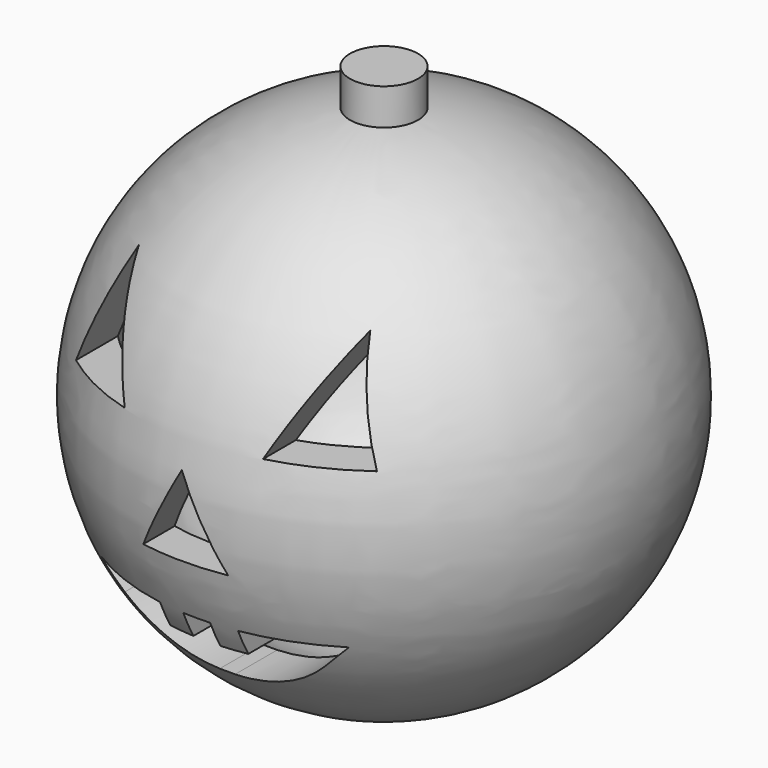
from build123d import *

# Parameters (mm, degrees)
F3_DEPTH = 50.8


# Not quite as in the source:
# - ends of sketch curves that miss each other by under 0.0002 mm in the source are joined


with BuildPart() as f1:
    # F0 (on Front) → F1 (revolve)
    with BuildSketch(Plane.XZ):
        with BuildLine():
            Line((-0.0036151696, -32.4747725203), (-0.0038838866, -38.0999998022))
            ThreePointArc((-0.0038838866, -38.0999998022), (38.0147276158, -2.5476258416), (5.0799988574, 37.7598146182))
            Line((5.0799988574, 37.7598146182), (5.0799988574, 43.18))
            Line((5.0799988574, 43.18), (-1.1426e-06, 43.18))
            Line((-1.1426e-06, 43.18), (-0.0005125311, 32.4747727174))
            ThreePointArc((-0.0005125311, 32.4747727174), (32.4747715418, -0.0015513193), (-0.0036151696, -32.4747725203))
        make_face()
    revolve(axis=Axis((-0.0037495281, 0, -35.2873861612), (4.777e-05, 0, 0.9999999989)))

    # F2 (on Front) → F3 (cut)
    with BuildSketch(Plane.XZ):
        Polygon((-10.317850841, 9.3550261232), (-17.2683447599, 23.8878782839), (-22.448848933, 9.2097846791), align=None)
        Polygon((6.3317239703, -6.6195321269), (-1.0035e-06, 5.4683093913), (-6.3317259774, -6.6195321269), (-1.0035e-06, -6.6195321269), align=None)
        with BuildLine():
            Line((-18.5189414894, -15.0686433726), (-14.959405017, -18.6930191949))
            ThreePointArc((-14.959405017, -18.6930191949), (-8.6349272642, -22.9699415744), (-1.1447285362, -24.4491328731))
            Line((-1.1447285362, -24.4491328731), (1.1447265291, -24.4491328731))
            ThreePointArc((1.1447265291, -24.4491328731), (8.6349252572, -22.9699415744), (14.9594030099, -18.6930191949))
            Line((14.9594030099, -18.6930191949), (18.5189414894, -15.0686433726))
            Line((18.5189414894, -15.0686433726), (5.8189414894, -15.0686433726))
            Line((5.8189414894, -15.0686433726), (5.8189414894, -18.8786433726))
            Line((5.8189414894, -18.8786433726), (2.0089414894, -18.8786433726))
            Line((2.0089414894, -18.8786433726), (2.0089414894, -15.0686433726))
            Line((2.0089414894, -15.0686433726), (-2.0089414894, -15.0686433726))
            Line((-2.0089414894, -15.0686433726), (-2.0089414894, -18.8786433726))
            Line((-2.0089414894, -18.8786433726), (-5.8189414894, -18.8786433726))
            Line((-5.8189414894, -18.8786433726), (-5.8189414894, -15.0686433726))
            Line((-5.8189414894, -15.0686433726), (-18.5189414894, -15.0686433726))
        make_face()
        Polygon((22.4488469259, 9.2097846791), (17.2683427529, 23.8878782839), (10.3178488339, 9.3550261232), align=None)
    extrude(amount=F3_DEPTH, mode=Mode.SUBTRACT)


solid = f1.part
